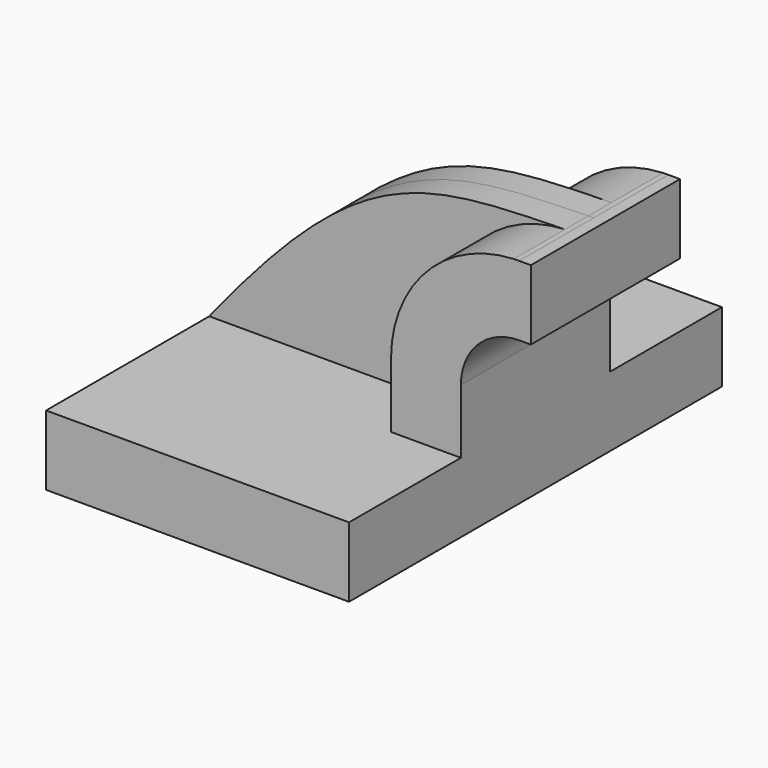
from build123d import *

# Parameters (mm, degrees)
F1_DEPTH = 63.5
F2_DEPTH = 25.4
F3_DEPTH = 7.9375


with BuildPart() as f1:
    # F0 (on Front) → F1 (new body, symmetric)
    with BuildSketch(Plane.XZ):
        Polygon((-41.275, -9.525), (41.275, -9.525), (41.275, 9.525), (22.225, 9.525), (-41.275, 9.525), align=None)
    extrude(amount=F1_DEPTH, both=True)

    # F0 (on Front) → F2 (join, symmetric)
    with BuildSketch(Plane.XZ):
        with BuildLine():
            Line((22.225, 9.525), (41.275, 9.525))
            Line((41.275, 9.525), (41.275, 27.0002))
            ThreePointArc((41.275, 27.0002), (45.9246798487, 38.2255201513), (57.15, 42.8752))
            Line((57.15, 42.8752), (60.325, 42.8752))
            Line((60.325, 42.8752), (60.325, 61.9252))
            Line((60.325, 61.9252), (57.15, 61.9252))
            add(Edge.make_bspline(
                [(55.6546739899, 61.8931738647), (56.1494536046, 61.9037814957), (56.6478649939, 61.9144247136), (57.15, 61.9252)],
                knots=[110.1378686708, 110.1378686708, 110.1378686708, 110.1378686708, 111.5045361635, 111.5045361635, 111.5045361635, 111.5045361635], degree=3))
            ThreePointArc((55.6546739899, 61.8931738647), (31.9311589689, 51.1614433879), (22.225, 27.0002))
            Line((22.225, 27.0002), (22.225, 9.525))
        make_face()
    extrude(amount=F2_DEPTH, both=True)

    # F0 (on Front) → F3 (join, symmetric)
    with BuildSketch(Plane.XZ):
        with BuildLine():
            add(Edge.make_bspline(
                [(-41.275, 9.525), (-0.5058915332, 60.4145856104), (15.7810598781, 61.0383193594), (55.6546739899, 61.8931738647)],
                knots=[0, 0, 0, 0, 110.1378686708, 110.1378686708, 110.1378686708, 110.1378686708], degree=3))
            Line((-41.275, 9.525), (22.225, 9.525))
            Line((22.225, 9.525), (22.225, 27.0002))
            ThreePointArc((22.225, 27.0002), (31.9311589689, 51.1614433879), (55.6546739899, 61.8931738647))
        make_face()
    extrude(amount=F3_DEPTH, both=True)


solid = f1.part
